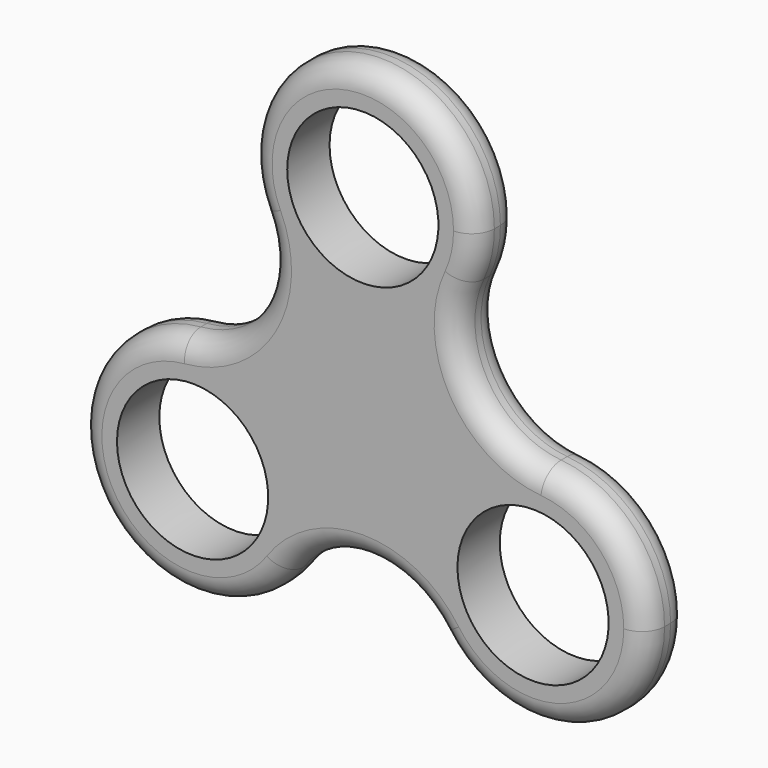
from build123d import *

# Parameters (mm, degrees)
F1_DEPTH = 3.5
F2_R     = 3
F4_D     = 20


with BuildPart() as f1:
    # F0 (on Front) → F1 (new body, symmetric)
    with BuildSketch(Plane.XZ):
        with BuildLine():
            ThreePointArc((13.59864, 19.66936), (14.64547, 22.758056), (15, 26))
            ThreePointArc((15, 26), (-3.241944, 40.64547), (-13.59864, 19.66936))
            ThreePointArc((-13.59864, 19.66936), (0, 11), (13.59864, 19.66936))
        make_face()
        with BuildLine():
            ThreePointArc((-7.51666, -13), (-12.386319, -1.937623), (-23.833485, 1.942087))
            ThreePointArc((-23.833485, 1.942087), (-35.507042, -20.5), (-10.234846, -21.611447))
            ThreePointArc((-10.234846, -21.611447), (-8.212339, -17.515129), (-7.51666, -13))
        make_face()
        with BuildLine():
            ThreePointArc((37.51666, -13), (33.579038, -2.869659), (23.833485, 1.942087))
            ThreePointArc((23.833485, 1.942087), (9.526279, -5.5), (10.234846, -21.611447))
            ThreePointArc((10.234846, -21.611447), (27.031789, -27.304321), (37.51666, -13))
        make_face()
        with BuildLine():
            ThreePointArc((13.59864, 19.66936), (0, 11), (-13.59864, 19.66936))
            ThreePointArc((-13.59864, 19.66936), (-14.105522, 8.143827), (-23.833485, 1.942087))
            ThreePointArc((-23.833485, 1.942087), (-12.386319, -1.937623), (-7.51666, -13))
            ThreePointArc((-7.51666, -13), (-8.212339, -17.515129), (-10.234846, -21.611447))
            ThreePointArc((-10.234846, -21.611447), (0, -16.287653), (10.234846, -21.611447))
            ThreePointArc((10.234846, -21.611447), (9.526279, -5.5), (23.833485, 1.942087))
            ThreePointArc((23.833485, 1.942087), (14.105522, 8.143827), (13.59864, 19.66936))
        make_face()
    extrude(amount=F1_DEPTH, both=True)

    # F2
    f2_edges = [f1.edges().sort_by_distance(p)[0] for p in [
        (-14.105522, -3.5, 8.143827),
        (-35.507042, -3.5, -20.5),
        (0, -3.5, -16.287653),
        (35.507042, -3.5, -20.5),
        (14.105522, -3.5, 8.143827),
        (0, -3.5, 41),
        (-14.105522, 3.5, 8.143827),
        (-35.507042, 3.5, -20.5),
        (0, 3.5, -16.287653),
        (35.507042, 3.5, -20.5),
        (14.105522, 3.5, 8.143827),
        (0, 3.5, 41),
    ]]
    fillet(f2_edges, radius=F2_R)

    # F4 (through all)
    with Locations(Plane.XZ.offset(3.5)):
        with Locations((0, 26), (-22.51666, -13), (22.51666, -13)):
            Hole(F4_D / 2)


solid = f1.part
